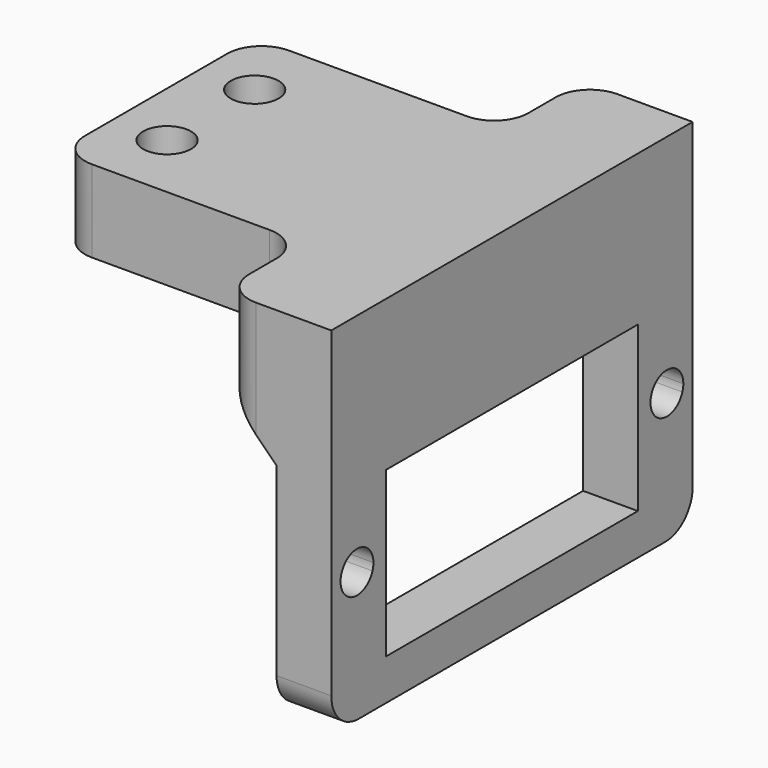
from build123d import *

# Parameters (mm, degrees)
F0_W      = 4
F0_H      = 18
F1_DEPTH  = 26
F0_W_2    = 7
F2_DEPTH  = 6
F3_W      = 4
F3_H      = 18
F4_DEPTH  = 15
F5_W      = 4
F5_H      = 18
F6_DEPTH  = 15
F7_W      = 11.5
F7_H      = 5.5
F7_H_2    = 6
F7_H_3    = 0.5
F8_DEPTH  = 25
F9_DEPTH  = 15
F10_DEPTH = 18
F11_DEPTH = 2
F12_DEPTH = 6
F13_DEPTH = 6
F14_DEPTH = 11
F15_W     = 9
F15_H     = 8
F16_DEPTH = 30
F18_D     = 3.5
F19_W     = 18
F19_H     = 6
F20_DEPTH = 9
F21_W     = 18
F21_H     = 6
F22_DEPTH = 9
F23_SIZE  = 4
F24_DEPTH = 1.5
F25_DEPTH = 1.5
F26_R     = 2.5


with BuildPart() as f1:
    # F0 (on Top) → F1 (new body)
    with BuildSketch(Plane.XY):
        with Locations((9, 9)):
            Rectangle(F0_W, F0_H)
    extrude(amount=-F1_DEPTH)

    # F0 (on Top) → F2 (join)
    with BuildSketch(Plane.XY):
        with Locations((3.5, 9)):
            Rectangle(F0_W_2, F0_H)
        with Locations((9, 9)):
            Rectangle(F0_W, F0_H)
    extrude(amount=-F2_DEPTH)

    # F3 (on face) → F4 (join)
    with BuildSketch(Plane.XZ):
        with Locations((9, -17)):
            Rectangle(F3_W, F3_H)
    extrude(amount=F4_DEPTH)

    # F5 (on face) → F6 (join)
    with BuildSketch(Plane(origin=(0, 18, 0), x_dir=(-1, 0, 0), z_dir=(0, 1, 0))):
        with Locations((-9, -17)):
            Rectangle(F5_W, F5_H)
    extrude(amount=F6_DEPTH)

    # F7 (on face) → F8 (cut)
    with BuildSketch(Plane.YZ.offset(11)):
        with Locations((3.25, -13.75)):
            Rectangle(F7_W, F7_H)
        with Locations((14.75, -13.75)):
            Rectangle(F7_W, F7_H)
        with BuildLine():
            Line((24.5675133947, -17), (21.7390862699, -17))
            ThreePointArc((21.7390862699, -17), (23.1532998323, -18), (24.5675133947, -17))
        make_face()
        with BuildLine():
            Line((24.6532998323, -16.5), (21.6532998323, -16.5))
            ThreePointArc((21.6532998323, -16.5), (21.6749019928, -16.7536529681), (21.7390862699, -17))
            Line((21.7390862699, -17), (24.5675133947, -17))
            ThreePointArc((24.5675133947, -17), (24.6316976718, -16.7536529681), (24.6532998323, -16.5))
        make_face()
        with BuildLine():
            ThreePointArc((24.6532998323, -16.5), (23.1532998323, -15), (21.6532998323, -16.5))
            Line((21.6532998323, -16.5), (24.6532998323, -16.5))
        make_face()
        with Locations((14.75, -20)):
            Rectangle(F7_W, F7_H_2)
        with Locations((14.75, -16.75)):
            Rectangle(F7_W, F7_H_3)
        with Locations((3.25, -20)):
            Rectangle(F7_W, F7_H_2)
        with Locations((3.25, -16.75)):
            Rectangle(F7_W, F7_H_3)
        with BuildLine():
            ThreePointArc((-3.6532998323, -16.5), (-5.1532998323, -15), (-6.6532998323, -16.5))
            Line((-6.6532998323, -16.5), (-3.6532998323, -16.5))
        make_face()
        with BuildLine():
            Line((-3.6532998323, -16.5), (-6.6532998323, -16.5))
            ThreePointArc((-6.6532998323, -16.5), (-6.6316976718, -16.7536529681), (-6.5675133947, -17))
            Line((-6.5675133947, -17), (-3.7390862699, -17))
            ThreePointArc((-3.7390862699, -17), (-3.6749019928, -16.7536529681), (-3.6532998323, -16.5))
        make_face()
        with BuildLine():
            Line((-3.7390862699, -17), (-6.5675133947, -17))
            ThreePointArc((-6.5675133947, -17), (-5.1532998323, -18), (-3.7390862699, -17))
        make_face()
    extrude(amount=-F8_DEPTH, mode=Mode.SUBTRACT)

    # F9 (add): a face of the model
    f9_faces = [f1.faces().sort_by_distance(p)[0] for p in [
        (0, 9, -3),
    ]]
    extrude(f9_faces, amount=F9_DEPTH)

    # F10 (add): a face of the model
    f10_faces = [f1.faces().sort_by_distance(p)[0] for p in [
        (-1.4634146341, 0, -3.1951219512),
    ]]
    extrude(f10_faces, amount=F10_DEPTH)

    # F11 (cut): a face of the model
    f11_faces = [f1.faces().sort_by_distance(p)[0] for p in [
        (-1.4634146341, 18, -3.1951219512),
    ]]
    extrude(f11_faces, amount=-F11_DEPTH, mode=Mode.SUBTRACT)

    # F12 (cut): a face of the model
    f12_faces = [f1.faces().sort_by_distance(p)[0] for p in [
        (9, -15, -17),
    ]]
    extrude(f12_faces, amount=-F12_DEPTH, mode=Mode.SUBTRACT)

    # F13 (cut): a face of the model
    f13_faces = [f1.faces().sort_by_distance(p)[0] for p in [
        (9, 33, -17),
    ]]
    extrude(f13_faces, amount=-F13_DEPTH, mode=Mode.SUBTRACT)

    # F14 (add): a face of the model
    f14_faces = [f1.faces().sort_by_distance(p)[0] for p in [
        (-1.4634146341, 16, -3.1951219512),
    ]]
    extrude(f14_faces, amount=F14_DEPTH)

    # F15 (on face) → F16 (cut)
    with BuildSketch(Plane.YZ.offset(11)):
        with Locations((-13.5, -4)):
            Rectangle(F15_W, F15_H)
    extrude(amount=-F16_DEPTH, mode=Mode.SUBTRACT)

    # F18 (through all)
    with Locations(Plane.XY):
        with Locations((-11, 13), (-11, 5)):
            Hole(F18_D / 2)

    # F19 (on face) → F20 (cut)
    with BuildSketch(Plane.XZ.offset(9)):
        with Locations((-6, -3)):
            Rectangle(F19_W, F19_H)
    extrude(amount=-F20_DEPTH, mode=Mode.SUBTRACT)

    # F21 (on face) → F22 (cut)
    with BuildSketch(Plane(origin=(0, 27, 0), x_dir=(-1, 0, 0), z_dir=(0, 1, 0))):
        with Locations((6, -3)):
            Rectangle(F21_W, F21_H)
    extrude(amount=-F22_DEPTH, mode=Mode.SUBTRACT)

    # F23
    f23_edges = [f1.edges().sort_by_distance(p)[0] for p in [
        (7, 9, -6),
    ]]
    chamfer(f23_edges, length=F23_SIZE)

    # F24 (cut): a face of the model
    f24_faces = [f1.faces().sort_by_distance(p)[0] for p in [
        (8.0980392157, -9, -10.9019607843),
    ]]
    extrude(f24_faces, amount=-F24_DEPTH, mode=Mode.SUBTRACT)

    # F25 (cut): a face of the model
    f25_faces = [f1.faces().sort_by_distance(p)[0] for p in [
        (8.0980392157, 27, -10.9019607843),
    ]]
    extrude(f25_faces, amount=-F25_DEPTH, mode=Mode.SUBTRACT)

    # F26
    f26_edges = [f1.edges().sort_by_distance(p)[0] for p in [
        (9, 25.5, -26),
        (3, 25.5, -3),
        (-15, 18, -3),
        (9, -7.5, -26),
        (3, -7.5, -3),
        (3, 0, -3),
        (3, 18, -3),
        (-15, 0, -3),
    ]]
    fillet(f26_edges, radius=F26_R)


solid = f1.part
